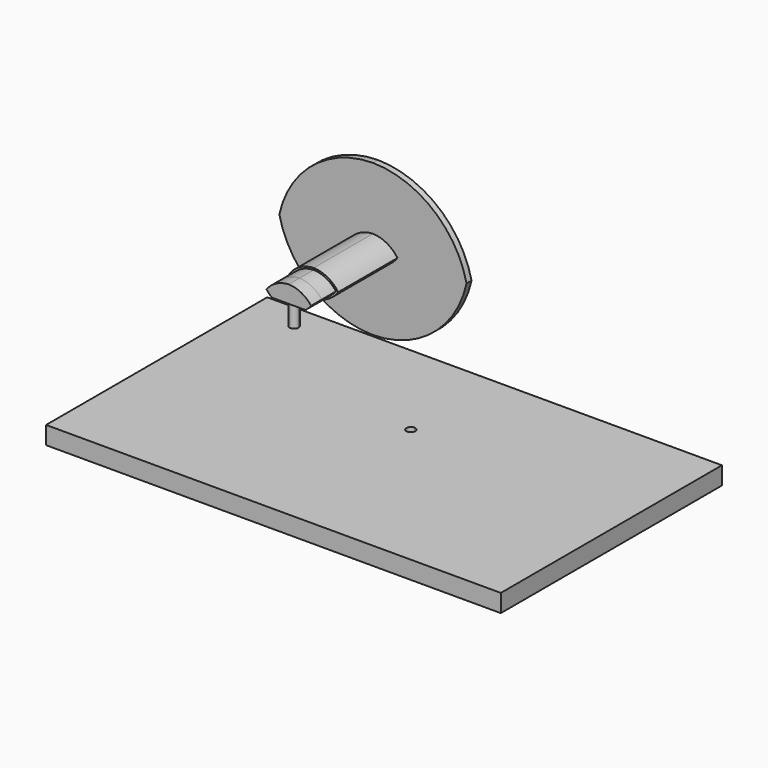
from build123d import *

# Parameters (mm, degrees)
F1_DEPTH        = 7
F3_DEPTH        = 83
F5_W            = 510
F5_H            = 310
F5_W_2          = 480
F5_H_2          = 273
F6_DEPTH        = 20
F7_DEPTH        = 15
F9_DEPTH        = 103
F11_DEPTH       = 15
F13_DEPTH       = 25
F15_DEPTH       = 8.42086
F16_TEXT_SIZE   = 27.2075436606
F16_TEXT_SIZE_2 = 171.1622220524


# Not quite as in the source:
# - Text() gives the source's letters only with a copy of the font that has no kerning and outlines rounded to 1/6400 em; it was checked with that copy


with BuildPart() as f1:
    # F0 (on Front) → F1 (new body)
    with BuildSketch(Plane.XZ):
        with BuildLine():
            ThreePointArc((0, 85), (-67.3032845966, 60.786410384), (-105, 0))
            Line((-105, 0), (0, 0))
            Line((0, 0), (0, 85))
        make_face()
        with BuildLine():
            Line((0, 0), (-105, 0))
            ThreePointArc((-105, 0), (-67.3032845966, -60.786410384), (0, -85))
            ThreePointArc((0, -85), (67.3032845966, -60.786410384), (105, 0))
            Line((105, 0), (0, 0))
        make_face()
        with BuildLine():
            Line((0, 85), (0, 0))
            Line((0, 0), (105, 0))
            ThreePointArc((105, 0), (67.3032845966, 60.786410384), (0, 85))
        make_face()
    extrude(amount=F1_DEPTH)

    # F2 (on face) → F3 (join)
    with BuildSketch(Plane.XZ.offset(7)):
        with BuildLine():
            ThreePointArc((0, 15), (-15.5139441376, 10.7338975856), (-27.5, 0))
            Line((-27.5, 0), (-25.0238620708, 0))
            ThreePointArc((-25.0238620708, 0), (-13.9634788205, 9.2936803356), (0, 12.9985192054))
            Line((0, 12.9985192054), (0, 15))
        make_face()
        with BuildLine():
            ThreePointArc((27.5, 0), (15.5139441376, 10.7338975856), (0, 15))
            Line((0, 15), (0, 12.9985192054))
            ThreePointArc((0, 12.9985192054), (13.9634788205, 9.2936803356), (25.0238620708, 0))
            Line((25.0238620708, 0), (27.5, 0))
        make_face()
        with BuildLine():
            Line((-25.0238620708, 0), (-27.5, 0))
            ThreePointArc((-27.5, 0), (-15.5139441376, -10.7338975856), (0, -15))
            ThreePointArc((0, -15), (15.5139441376, -10.7338975856), (27.5, 0))
            Line((27.5, 0), (25.0238620708, 0))
            ThreePointArc((25.0238620708, 0), (13.9634788205, -9.2936803356), (0, -12.9985192054))
            ThreePointArc((0, -12.9985192054), (-13.9634788205, -9.2936803356), (-25.0238620708, 0))
        make_face()
    extrude(amount=F3_DEPTH)


with BuildPart() as f6:
    # F5 (on offset) → F6 (new body)
    with BuildSketch(Plane.XY.offset(-200)):
        with Locations((0, 8.5)):
            Rectangle(F5_W, F5_H)
        Rectangle(F5_W_2, F5_H_2, mode=Mode.SUBTRACT)
    extrude(amount=-F6_DEPTH)

    # F5 (on offset) → F7 (join)
    with BuildSketch(Plane.XY.offset(-200)):
        Rectangle(F5_W_2, F5_H_2)
    extrude(amount=-F7_DEPTH)

    # F14 (on face) → F15 (cut)
    with BuildSketch(Plane.XY.offset(-200)):
        with BuildLine():
            ThreePointArc((5, 46.1195968091), (3.5355339059, 49.6551307151), (0, 51.1195968091))
            ThreePointArc((0, 51.1195968091), (-3.5355339059, 42.5840629032), (5, 46.1195968091))
        make_face()
    extrude(amount=-F15_DEPTH, mode=Mode.SUBTRACT)

    # F16 (on offset) → F17 (join, up to the next surface of F6)
    with BuildSketch(Plane(origin=(0, 0, -225), x_dir=(1, 0, 0), z_dir=(0, 0, -1))):
        with Locations((-25.9571790194, -161.4123878623)):
            Text('KDU', F16_TEXT_SIZE, font='Open Sans', font_style=FontStyle.BOLD, text_align=(TextAlign.LEFT, TextAlign.BOTTOM))
        with Locations((-175, -57.439165165)):
            Text('KDU', F16_TEXT_SIZE_2, font='Open Sans', text_align=(TextAlign.LEFT, TextAlign.BOTTOM))
    extrude(until=Until.NEXT, dir=(0, 0, 1))


with BuildPart() as f9:
    # F9 (new): a face of the model
    f9_faces = [f1.part.faces().sort_by_distance(p)[0] for p in [
        (0, -7, 0),
    ]]
    extrude(f9_faces, amount=F9_DEPTH)


with BuildPart() as f11:
    # F10 (on face) → F11 (new body)
    with BuildSketch(Plane.XZ.offset(110)):
        with BuildLine():
            ThreePointArc((-25.0238620708, 0), (-22.0941052007, -3.3445691771), (-18.7429838516, -6.2668292616))
            Line((-18.7429838516, -6.2668292616), (18.7429838516, -6.2668292616))
            ThreePointArc((18.7429838516, -6.2668292616), (22.0941052007, -3.3445691771), (25.0238620708, 0))
            ThreePointArc((25.0238620708, 0), (13.9634788205, 9.2936803356), (0, 12.9985192054))
            ThreePointArc((0, 12.9985192054), (-13.9634788205, 9.2936803356), (-25.0238620708, 0))
        make_face()
    extrude(amount=F11_DEPTH)

    # F12 (on face) → F13 (join)
    with BuildSketch(Plane(origin=(0, 0, -6.2668292616), x_dir=(1, 0, 0), z_dir=(0, 0, -1))):
        with BuildLine():
            ThreePointArc((5, 117.5), (-3.5355377121, 121.0355300997), (1.07656e-05, 112.5))
            ThreePointArc((1.07656e-05, 112.5), (3.5355377121, 113.9644699003), (5, 117.5))
        make_face()
    extrude(amount=F13_DEPTH)


solid = Compound([f1.part, f6.part, f9.part, f11.part])
